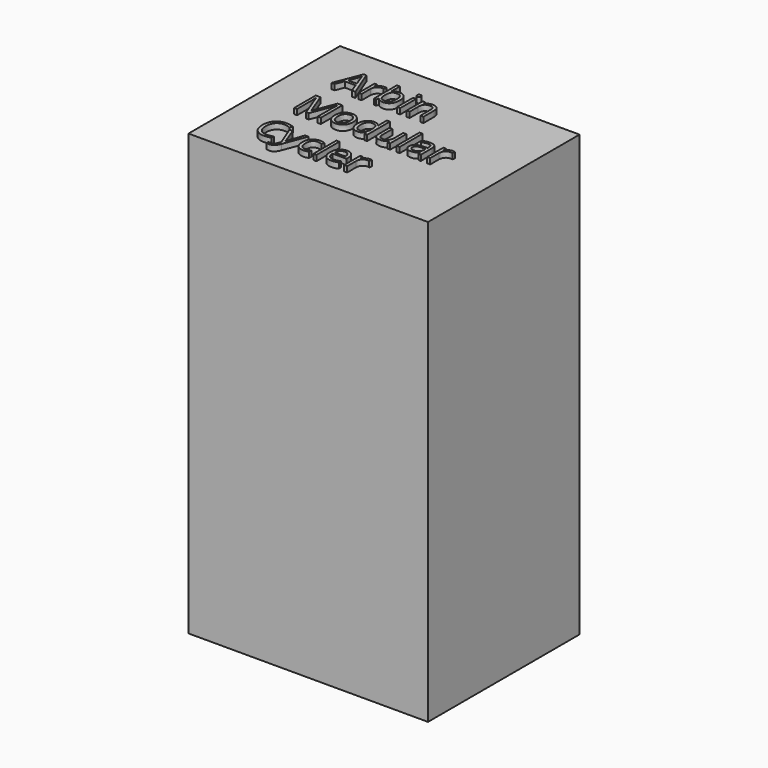
from build123d import *

# Parameters (mm, degrees)
F0_W         = 1092.2
F0_H         = 863.6
F1_DEPTH     = 2006.6
F2_TEXT_SIZE = 171.6910550992
F3_DEPTH     = 25.4


# Not quite as in the source:
# - Text() gives the source's letters only with a copy of the font that has no kerning and outlines rounded to 1/6400 em; it was checked with that copy


with BuildPart() as f1:
    # F0 (on Top) → F1 (new body)
    with BuildSketch(Plane.XY):
        Rectangle(F0_W, F0_H)
    extrude(amount=F1_DEPTH)

    # F2 (on face) → F3 (join)
    with BuildSketch(Plane.XY.offset(2006.6)):
        with Locations((-362.0666265488, 153.2542705536)):
            Text('Arbin', F2_TEXT_SIZE, font='Open Sans', text_align=(TextAlign.LEFT, TextAlign.BOTTOM))
        with Locations((-362.0666265488, -80.2455643813)):
            Text('Modular', F2_TEXT_SIZE, font='Open Sans', text_align=(TextAlign.LEFT, TextAlign.BOTTOM))
        with Locations((-362.0666265488, -313.7453993162)):
            Text('Cycler', F2_TEXT_SIZE, font='Open Sans', text_align=(TextAlign.LEFT, TextAlign.BOTTOM))
    extrude(amount=F3_DEPTH)


solid = f1.part
